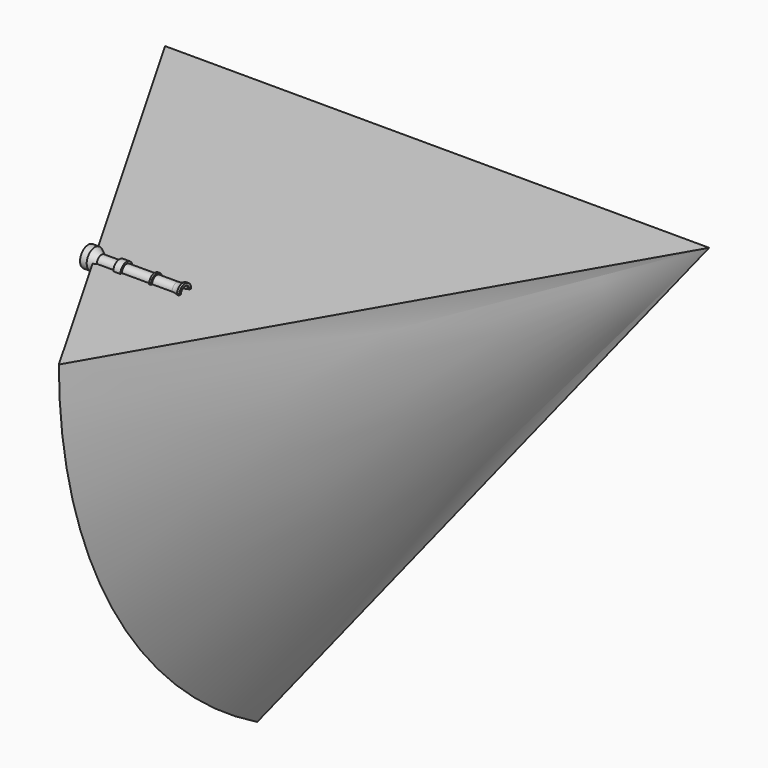
from build123d import *

# Parameters (mm, degrees)
F5_T     = 1
F7_ANGLE = 61.6159971065


# Not quite as in the source:
# - a fillet or chamfer that OpenCascade refuses, or shapes differently, is made with other operations: its cross-section is extruded or revolved along the edge and cut away or added
# - a feature of the source that left no trace in its solid (it failed there, or was rolled back) is left out
# - a shell that OpenCascade refuses in one call is made with other operations: the cavity is built on its own and cut out


with BuildPart() as f1:
    # F0 (on Front) → F1 (revolve)
    with BuildSketch(Plane.XZ):
        Polygon((-42, 4.4344547205), (-42, 0), (0, 0), (0, 3.3141644672), (-0.939540565, 3.3141644672), (-0.939540565, 2.5), (-12.3243089765, 2.5), (-12.3243089765, 3.1194374897), (-13.1681719795, 3.1194374897), (-13.1681719795, 2.5), (-25.396803394, 2.5), (-25.396803394, 3.3141644672), (-28.4831486642, 3.3141644672), (-28.4831486642, 2.5), (-36.2527966499, 2.5), (-39.1136556864, 4.4344547205), align=None)
    revolve(axis=Axis((-21, 0, 0), (1, 0, 0)))

    # F4: fillet of radius 5 on 1 edges, made by hand

    # F4_s1 → F4_t2 (revolve)
    with BuildSketch(Plane.XZ):
        with BuildLine():
            ThreePointArc((-0.939540565, 3.3141644672), (-2.2475981784, 2.7078617683), (-3.6742765472, 2.5))
            Line((-3.6742765472, 2.5), (-0.939540565, 2.5))
            Line((-0.939540565, 2.5), (-0.939540565, 3.3141644672))
        make_face()
    revolve(axis=Axis((-0.939540565, 0, 0), (1, 0, 0)))

    # F5: shell of thickness 1, made by hand


with BuildPart() as f5_core1:
    # F5_t2: copy of F1
    add(f1.part)

    # the walls: a layer under each face that stays
    f5_faces = [f5_core1.faces().sort_by_distance(p)[0] for p in [
        (-40.5568278432, 0, -4.4344547205),
        (-37.6832261682, 0, -3.4672273602),
        (-32.3679726571, 0, -2.5),
        (-28.4831486642, 2.2094429781, -2.2094429781),
        (-26.9399760291, 0, -3.3141644672),
        (-25.396803394, 2.2094429781, 2.2094429781),
        (-19.2824876867, 0, -2.5),
        (-13.1681719795, 2.0796249931, -2.0796249931),
        (-12.746240478, 0, -3.1194374897),
        (-12.3243089765, 2.0796249931, 2.0796249931),
        (-7.9992927619, 0, -2.5),
        (-2.2475981784, 0, -2.7078617683),
        (-0.4697702825, 0, -3.3141644672),
    ]]
    thicken(f5_faces, amount=-F5_T, mode=Mode.SUBTRACT)

    # F5_s3 → F5_t4 (revolve, cut)
    with BuildSketch(Plane.XZ):
        Polygon((-36.2471952097, 2.5182839524), (-36.8129406711, 1.6716047589), (-36.5591549299, 1.5), (-36.2527966499, 1.5), align=None)
    revolve(axis=Axis((-36.2527966499, 0, 0), (1, 0, 0)), mode=Mode.SUBTRACT)

    # F5_s5 → F5_t6 (revolve, cut)
    with BuildSketch(Plane.XZ):
        Polygon((-28.4931486642, 2.51), (-28.4831486642, 1.5), (-27.4831486642, 1.5), (-27.4831486642, 2.5), align=None)
    revolve(axis=Axis((-28.4831486642, 0, 0), (1, 0, 0)), mode=Mode.SUBTRACT)

    # F5_s7 → F5_t8 (revolve, cut)
    with BuildSketch(Plane.XZ):
        Polygon((-25.386803394, 2.51), (-26.396803394, 2.5), (-26.396803394, 1.5), (-25.396803394, 1.5), align=None)
    revolve(axis=Axis((-25.396803394, 0, 0), (1, 0, 0)), mode=Mode.SUBTRACT)

    # F5_s9 → F5_t10 (revolve, cut)
    with BuildSketch(Plane.XZ):
        Polygon((-13.1781719795, 2.51), (-13.1681719795, 1.5), (-12.1681719795, 1.5), (-12.1681719795, 2.5), align=None)
    revolve(axis=Axis((-13.1681719795, 0, 0), (1, 0, 0)), mode=Mode.SUBTRACT)

    # F5_s11 → F5_t12 (revolve, cut)
    with BuildSketch(Plane.XZ):
        Polygon((-12.3143089765, 2.51), (-13.3243089765, 2.5), (-13.3243089765, 1.5), (-12.3243089765, 1.5), align=None)
    revolve(axis=Axis((-12.3243089765, 0, 0), (1, 0, 0)), mode=Mode.SUBTRACT)


with BuildPart() as f1_1:
    add(f1.part)

    # what is left inside the walls is the cavity
    f5_cavity = [f5_core1.part.solids().sort_by_distance(p)[0] for p in [
        (-18.822628, 0, -1.49),
    ]]
    add(f5_cavity, mode=Mode.SUBTRACT)

    # F6 (on Top) → F7 (revolve)
    with BuildSketch(Plane.XY):
        Polygon((-0.2392299093, -68.1274962625), (118.1739337362, 136.1414027413), (-117.9347038269, 136.5557610989), align=None)
    revolve(axis=Axis((0.1196149546, 136.3485819201, 0), (0.9999984601, -0.0017549452, 0)), revolution_arc=F7_ANGLE)


solid = f1_1.part
